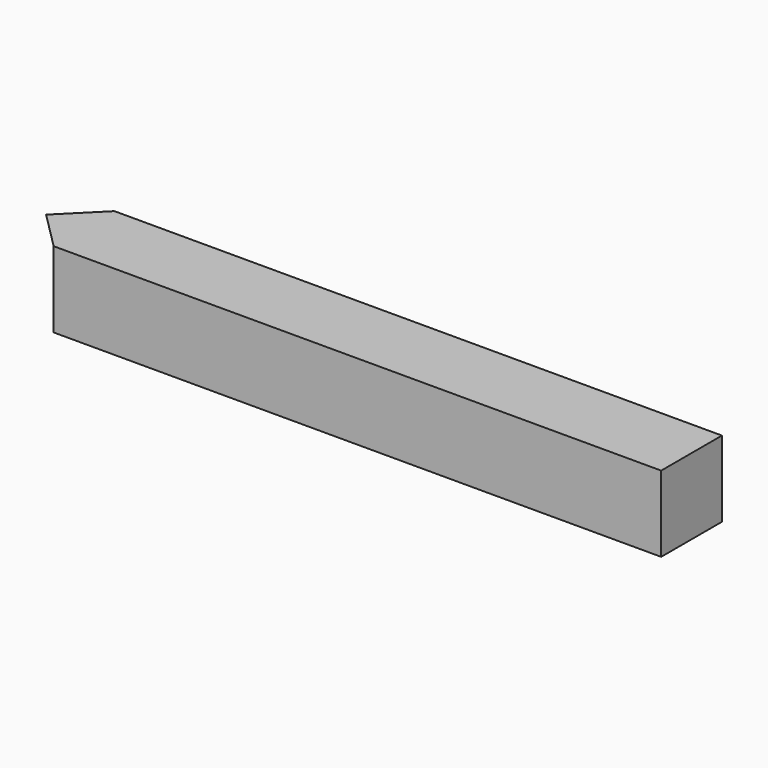
from build123d import *

# Parameters (mm, degrees)
F0_W     = 76.2
F0_H     = 9.525
F1_DEPTH = 9.525
F2_DEPTH = 9.525
F2_TAPER = 12


with BuildPart() as f1:
    # F0 (on Top) → F1 (new body)
    with BuildSketch(Plane.XY):
        with Locations((38.1, -4.7625)):
            Rectangle(F0_W, F0_H)
    extrude(amount=-F1_DEPTH)

    # F0 (on Top) → F2 (join)
    with BuildSketch(Plane.XY):
        with Locations((38.1, -4.7625)):
            Rectangle(F0_W, F0_H)
        Polygon((0, -9.525), (0, 0), (-4.7625, -4.7625), align=None)
    extrude(amount=-F2_DEPTH, taper=F2_TAPER)


solid = f1.part
